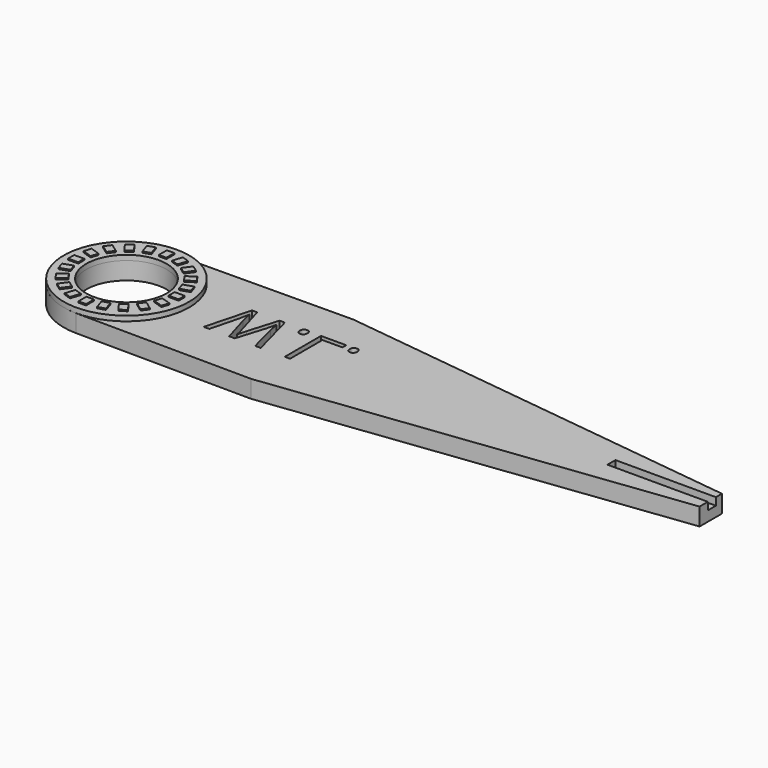
from build123d import *

# Parameters (mm, degrees)
F0_R         = 8
F1_DEPTH     = 3.5
F2_R         = 12.5
F2_R_2       = 8
F3_DEPTH     = 1
F4_W         = 1.5
F4_H         = 2
F4_W_2       = 2
F4_H_2       = 1.5
F5_DEPTH     = 0.25
F7_TEXT_SIZE = 12.6460647961
F8_DEPTH     = 25
F6_W         = 20
F6_H         = 2
F9_DEPTH     = 1.5


# Not quite as in the source:
# - Text() gives the source's letters only with a copy of the font that has no kerning and outlines rounded to 1/6400 em; it was checked with that copy


with BuildPart() as f1:
    # F0 (on Top) → F1 (new body)
    with BuildSketch(Plane.XY):
        with BuildLine():
            ThreePointArc((0, -12.5), (8.8388347648, -8.8388347648), (12.5, 0))
            ThreePointArc((12.5, 0), (8.8388347648, 8.8388347648), (0, 12.5))
            ThreePointArc((0, 12.5), (-12.5, 0), (0, -12.5))
        make_face()
        Circle(F0_R, mode=Mode.SUBTRACT)
        with BuildLine():
            ThreePointArc((0, 12.5), (8.8388347648, 8.8388347648), (12.5, 0))
            ThreePointArc((12.5, 0), (8.8388347648, -8.8388347648), (0, -12.5))
            Line((0, -12.5), (34.9989484294, -12.7713094819))
            Line((34.9989484294, -12.7713094819), (116.387732864, -2.7780233227))
            Line((116.387732864, -2.7780233227), (116.387732864, 2.7780233227))
            Line((116.387732864, 2.7780233227), (34.9989484294, 12.7713094819))
            Line((34.9989484294, 12.7713094819), (0, 12.5))
        make_face()
    extrude(amount=F1_DEPTH)

    # F7 (on face) → F8 (cut, symmetric)
    with BuildSketch(Plane(origin=(0, 0, 0), x_dir=(1, 0, 0), z_dir=(0, 0, -1))):
        with Locations((18.1754138321, -5.3274910897)):
            Text('W.L.', F7_TEXT_SIZE, font='Open Sans', text_align=(TextAlign.LEFT, TextAlign.BOTTOM))
    extrude(amount=F8_DEPTH, both=True, mode=Mode.SUBTRACT)

    # F6 (on face) → F9 (cut)
    with BuildSketch(Plane.XY.offset(3.5)):
        with Locations((106.387732864, 0.2780233227)):
            Rectangle(F6_W, F6_H)
    extrude(amount=-F9_DEPTH, mode=Mode.SUBTRACT)


with BuildPart() as f3:
    # F2 (on face) → F3 (new body)
    with BuildSketch(Plane.XY.offset(3.5)):
        Circle(F2_R)
        Circle(F2_R_2, mode=Mode.SUBTRACT)
    extrude(amount=F3_DEPTH)

    # F4 (on face) → F5 (join)
    with BuildSketch(Plane.XY.offset(4.5)):
        with Locations((0, 10)):
            Rectangle(F4_W, F4_H)
        Polygon((-2.6858945509, 10.693384425), (-4.1124793253, 10.2298589335), (-3.4944453366, 8.3277459009), (-2.0678605622, 8.7912713924), align=None)
        Polygon((-5.8588750294, 9.3400258773), (-7.072400521, 8.4583479989), (-5.8968300164, 6.8403140102), (-4.6833045249, 7.7219918886), align=None)
        Polygon((-8.4583479989, 7.072400521), (-9.3400258773, 5.8588750294), (-7.7219918886, 4.6833045249), (-6.8403140102, 5.8968300164), align=None)
        Polygon((-10.2298589335, 4.1124793253), (-10.693384425, 2.6858945509), (-8.7912713924, 2.0678605622), (-8.3277459009, 3.4944453366), align=None)
        with Locations((-10, 0)):
            Rectangle(F4_W_2, F4_H_2)
        Polygon((-10.693384425, -2.6858945509), (-10.2298589335, -4.1124793253), (-8.3277459009, -3.4944453366), (-8.7912713924, -2.0678605622), align=None)
        Polygon((-9.3400258773, -5.8588750294), (-8.4583479989, -7.072400521), (-6.8403140102, -5.8968300164), (-7.7219918886, -4.6833045249), align=None)
        Polygon((-7.072400521, -8.4583479989), (-5.8588750294, -9.3400258773), (-4.6833045249, -7.7219918886), (-5.8968300164, -6.8403140102), align=None)
        Polygon((-4.1124793253, -10.2298589335), (-2.6858945509, -10.693384425), (-2.0678605622, -8.7912713924), (-3.4944453366, -8.3277459009), align=None)
        with Locations((0, -10)):
            Rectangle(F4_W, F4_H)
        Polygon((2.6858945509, -10.693384425), (4.1124793253, -10.2298589335), (3.4944453366, -8.3277459009), (2.0678605622, -8.7912713924), align=None)
        Polygon((5.8588750294, -9.3400258773), (7.072400521, -8.4583479989), (5.8968300164, -6.8403140102), (4.6833045249, -7.7219918886), align=None)
        Polygon((8.4583479989, -7.072400521), (9.3400258773, -5.8588750294), (7.7219918886, -4.6833045249), (6.8403140102, -5.8968300164), align=None)
        Polygon((10.2298589335, -4.1124793253), (10.693384425, -2.6858945509), (8.7912713924, -2.0678605622), (8.3277459009, -3.4944453366), align=None)
        with Locations((10, 0)):
            Rectangle(F4_W_2, F4_H_2)
        Polygon((10.693384425, 2.6858945509), (10.2298589335, 4.1124793253), (8.3277459009, 3.4944453366), (8.7912713924, 2.0678605622), align=None)
        Polygon((9.3400258773, 5.8588750294), (8.4583479989, 7.072400521), (6.8403140102, 5.8968300164), (7.7219918886, 4.6833045249), align=None)
        Polygon((7.072400521, 8.4583479989), (5.8588750294, 9.3400258773), (4.6833045249, 7.7219918886), (5.8968300164, 6.8403140102), align=None)
        Polygon((4.1124793253, 10.2298589335), (2.6858945509, 10.693384425), (2.0678605622, 8.7912713924), (3.4944453366, 8.3277459009), align=None)
    extrude(amount=F5_DEPTH)


solid = Compound([f1.part, f3.part])
